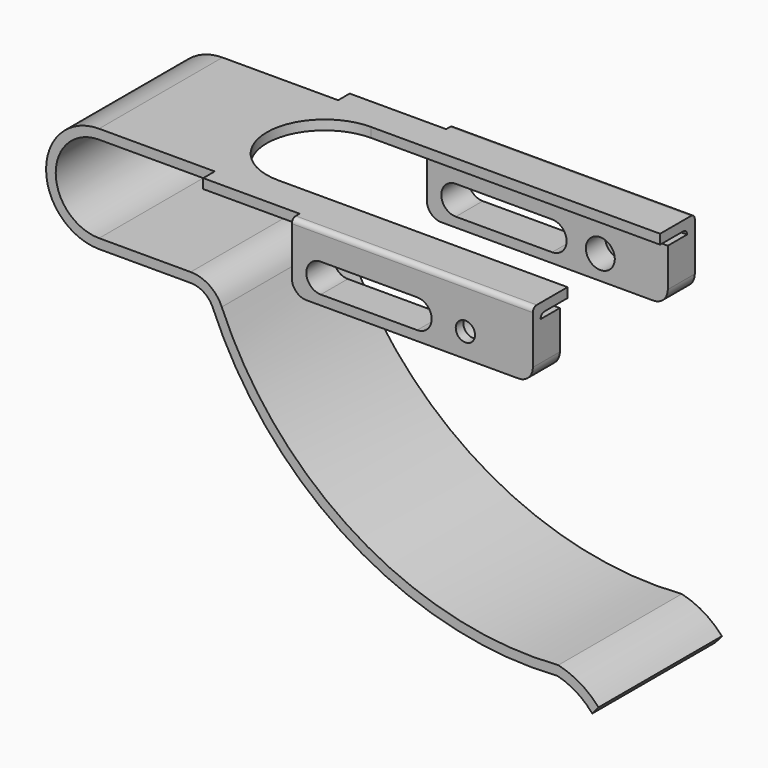
from build123d import *

# Parameters (mm, degrees)
F1_DEPTH       = 16
F2_W           = 70
F2_H           = 3
F3_DEPTH       = 2
F4_W           = 50
F4_H           = 14
F5_DEPTH       = 2
F6_R           = 1
F9_DEPTH       = 2
F11_DEPTH      = 21.001
F11_DEPTH_BACK = 25
F13_D          = 4
F14_W          = 50
F14_H          = 11
F14_R          = 3
F15_DEPTH      = 5
F16_R          = 3


# Not quite as in the source:
# - a pattern or mirror of a feature is missing from the dataset's text; its kind, count and spacing are read off the source's solid


with BuildPart() as f1:
    # F0 (on Front) → F1 (new body)
    with BuildSketch(Plane.XZ):
        with BuildLine():
            ThreePointArc((0, -9), (-9, 0), (0, 9))
            Line((0, 9), (94, 9))
            Line((94, 9), (94, 11))
            Line((94, 11), (0, 11))
            ThreePointArc((0, 11), (-11, 0), (0, -11))
            Line((0, -11), (19, -11))
            ThreePointArc((19, -11), (21.7681124643, -11.8361612201), (23.6103896104, -14.064978646))
            ThreePointArc((23.6103896104, -14.064978646), (52.3002338891, -47.5417473959), (95.1260447976, -58.0179647813))
            ThreePointArc((95.1260447976, -58.0179647813), (99.0798371754, -59.7246197028), (102.3278575446, -62.552252789))
            Line((102.3278575446, -62.552252789), (103.6303522873, -61))
            ThreePointArc((103.6303522873, -61), (99.852279938, -57.8519370421), (95.2965735981, -56))
            ThreePointArc((95.2965735981, -56), (53.4811996085, -45.9198240056), (25.4545454545, -13.2909701044))
            ThreePointArc((25.4545454545, -13.2909701044), (22.87535745, -10.1706257081), (19, -9))
            Line((19, -9), (0, -9))
        make_face()
    extrude(amount=F1_DEPTH)

    # F2 (on face) → F3 (join)
    with BuildSketch(Plane.XY.offset(11)):
        with Locations((59, -17.5)):
            Rectangle(F2_W, F2_H)
    extrude(amount=-F3_DEPTH)

    # F4 (on face) → F5 (join)
    with BuildSketch(Plane.XZ.offset(19)):
        with Locations((69, 4)):
            Rectangle(F4_W, F4_H)
    extrude(amount=F5_DEPTH)

    # F6
    f6_edges = [f1.edges().sort_by_distance(p)[0] for p in [
        (69, -21, 11),
        (69, -19, 9),
    ]]
    fillet(f6_edges, radius=F6_R)

    # F7: F1 across plane


with BuildPart() as f1_1:
    add(f1.part)
    add(f1.part.mirror(Plane.XZ))

    # F8 (on face) → F9 (cut)
    with BuildSketch(Plane.XY.offset(11)):
        with BuildLine():
            Line((94, 12), (34, 12))
            ThreePointArc((34, 12), (22, 0), (34, -12))
            Line((34, -12), (94, -12))
            Line((94, -12), (94, 12))
        make_face()
    extrude(amount=-F9_DEPTH, mode=Mode.SUBTRACT)

    # F10 (on Front) → F11 (cut, two sides)
    with BuildSketch(Plane.XZ) as f11_sk:
        with BuildLine():
            ThreePointArc((50, 5), (47, 2), (50, -1))
            Line((50, -1), (70, -1))
            ThreePointArc((70, -1), (73, 2), (70, 5))
            Line((70, 5), (50, 5))
        make_face()
    extrude(amount=-F11_DEPTH, mode=Mode.SUBTRACT)
    extrude(f11_sk.sketch, amount=F11_DEPTH_BACK, mode=Mode.SUBTRACT)

    # F13 (through all)
    with Locations(Plane.XZ.offset(21)):
        with Locations((80, 2)):
            Hole(F13_D / 2)

    # F14 (on face) → F15 (join)
    with BuildSketch(Plane(origin=(0, -19, 0), x_dir=(-1, 0, 0), z_dir=(0, 1, 0))):
        with Locations((-69, 2.5)):
            Rectangle(F14_W, F14_H)
        with Locations((-80, 2)):
            Circle(F14_R, mode=Mode.SUBTRACT)
        with BuildLine():
            Line((-70, 5), (-50, 5))
            ThreePointArc((-50, 5), (-47, 2), (-50, -1))
            Line((-50, -1), (-70, -1))
            ThreePointArc((-70, -1), (-73, 2), (-70, 5))
        make_face(mode=Mode.SUBTRACT)
    f15 = extrude(amount=F15_DEPTH)

    # F15_copies: F15 across plane
    add(f15.mirror(Plane.ZX))

    # F16
    f16_edges = [f1_1.edges().sort_by_distance(p)[0] for p in [
        (44, -17.5, -3),
        (94, -17.5, -3),
        (44, 17.5, -3),
        (94, 17.5, -3),
    ]]
    fillet(f16_edges, radius=F16_R)


solid = f1_1.part
